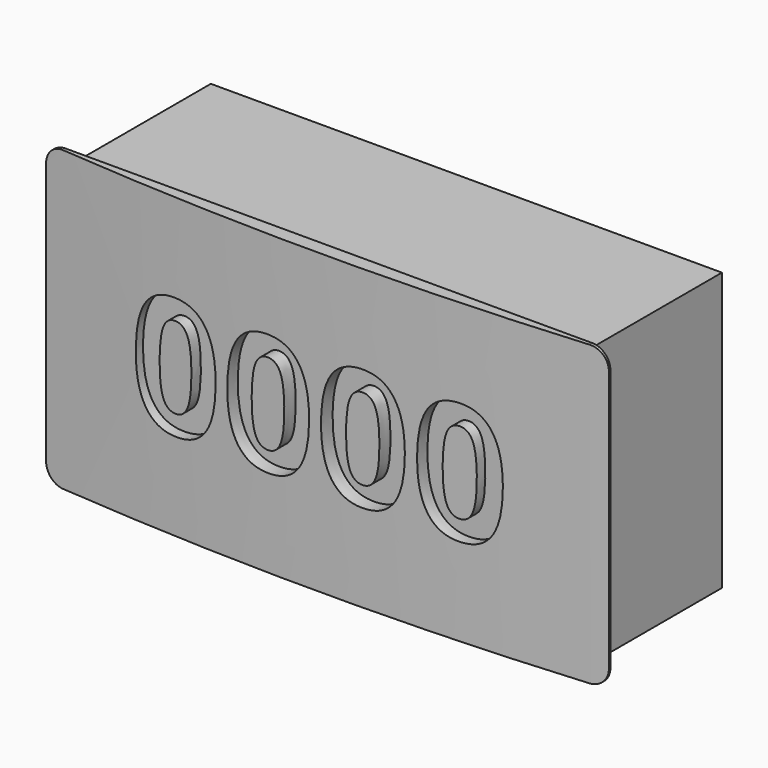
from build123d import *

# Parameters (mm, degrees)
F0_W         = 79.0956
F0_H         = 41.91
F1_DEPTH     = 2.032
F2_R         = 444.5
F3_DEPTH     = 50.8
F4_W         = 71.8312
F4_H         = 39.0144
F5_DEPTH     = 24.13
F6_W         = 14.6558
F6_H         = 5.715
F7_DEPTH     = 1.016
F8_TEXT_SIZE = 23.3421177107
F9_DEPTH     = 4.2418
F10_R        = 2.54


# Not quite as in the source:
# - Text() gives the source's letters only with a copy of the font that has no kerning and outlines rounded to 1/6400 em; it was checked with that copy


with BuildPart() as f1:
    # F0 (on Front) → F1 (new body)
    with BuildSketch(Plane.XZ):
        Rectangle(F0_W, F0_H)
    extrude(amount=F1_DEPTH)

    # F2 (on face) → F3 (intersect)
    with BuildSketch(Plane(origin=(0, 0, -20.955), x_dir=(1, 0, 0), z_dir=(0, 0, -1))):
        with Locations((0, -442.468)):
            Circle(F2_R)
    extrude(amount=-F3_DEPTH, mode=Mode.INTERSECT)

    # F4 (on face) → F5 (join)
    with BuildSketch(Plane(origin=(0, 0, 0), x_dir=(-1, 0, 0), z_dir=(0, 1, 0))):
        Rectangle(F4_W, F4_H)
    extrude(amount=F5_DEPTH)

    # F6 (on face) → F7 (join)
    with BuildSketch(Plane(origin=(0, 0, -19.5072), x_dir=(1, 0, 0), z_dir=(0, 0, -1))):
        with Locations((0, -12.3825)):
            Rectangle(F6_W, F6_H)
    extrude(amount=F7_DEPTH)

    # F8 (on Front) → F9 (cut)
    with BuildSketch(Plane.XZ):
        with Locations((-26.9875, -8.4031623758)):
            Text('0000', F8_TEXT_SIZE, font='Open Sans', font_style=FontStyle.BOLD, text_align=(TextAlign.LEFT, TextAlign.BOTTOM))
    extrude(amount=F9_DEPTH, mode=Mode.SUBTRACT)

    # F10
    f10_edges = [f1.edges().sort_by_distance(p)[0] for p in [
        (-39.5478, -0.134596, 20.955),
        (39.5478, -0.134596, 20.955),
        (39.5478, -0.134596, -20.955),
        (-39.5478, -0.134596, -20.955),
    ]]
    fillet(f10_edges, radius=F10_R)


solid = f1.part
